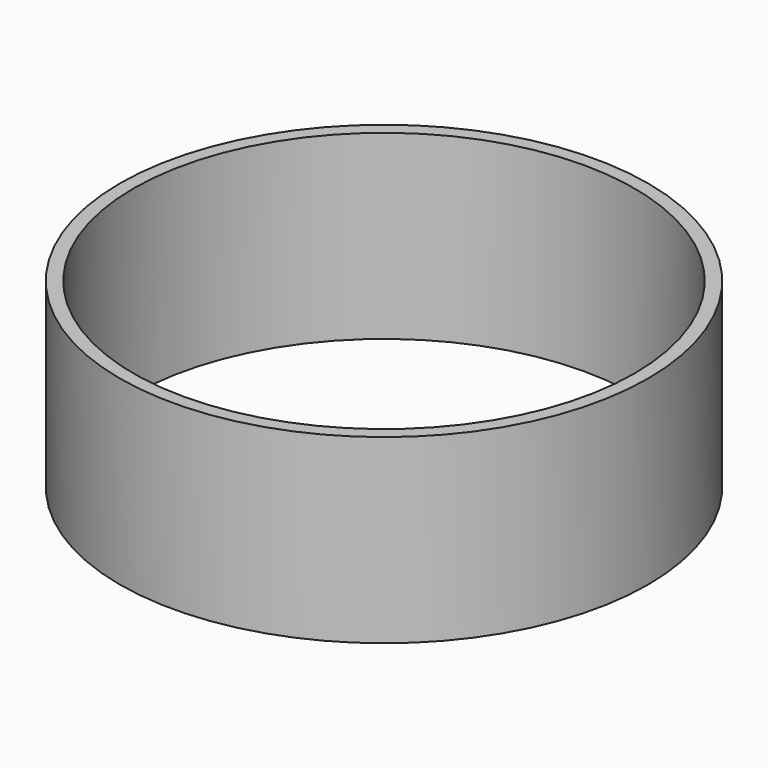
from build123d import *

# Parameters (mm, degrees)
F0_W = 6.3
F0_H = 83.9970919721


# Not quite as in the source:
# - a feature names something its author has since deleted; it is built from what else it names


with BuildPart() as f1:
    # F0 (on Front) → F1 (revolve)
    with BuildSketch(Plane.XZ):
        with Locations((-119.1, -30.1424739006)):
            Rectangle(F0_W, F0_H)
    revolve(axis=Axis((0, 0, -33.1439279145), (0, 0, -1)))


solid = f1.part
